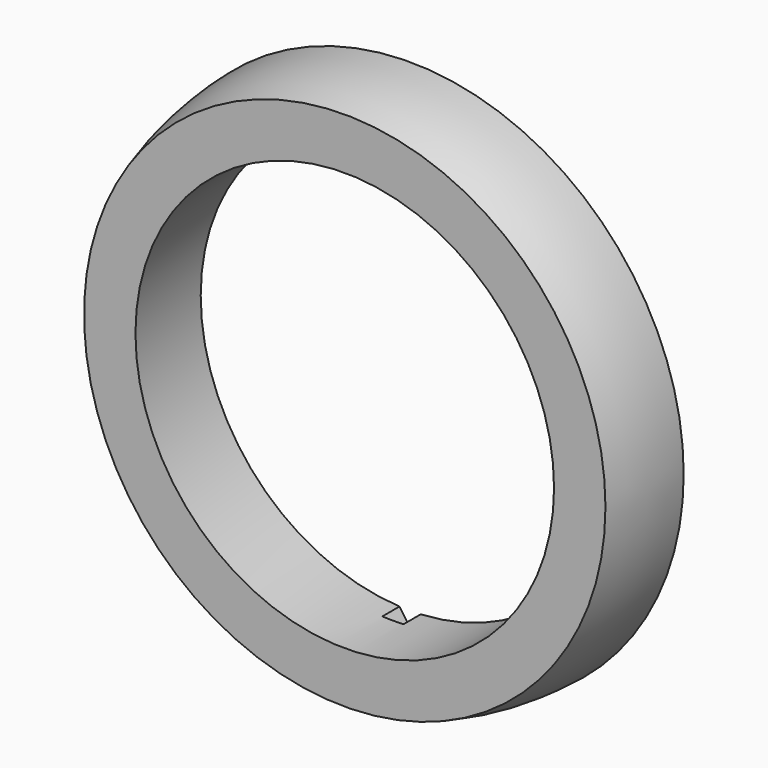
from build123d import *

# Parameters (mm, degrees)
F3_DEPTH = 10


with BuildPart() as f1:
    # F0 (on Top) → F1 (revolve)
    with BuildSketch(Plane.XY):
        with BuildLine():
            Line((97.4973875252, -38.8161949813), (121.4477377606, -38.8161949813))
            ThreePointArc((121.4477377606, -38.8161949813), (120.5697284263, -19.6675259883), (117.0955747366, -0.8161949813))
            Line((117.0955747366, -0.8161949813), (97.4973875252, -0.8161949813))
            Line((97.4973875252, -0.8161949813), (97.4973875252, -38.8161949813))
        make_face()
        with BuildLine():
            ThreePointArc((117.0955747366, -0.8161949813), (120.5697284263, -19.6675259883), (121.4477377606, -38.8161949813))
            ThreePointArc((121.4477377606, -38.8161949813), (125.914331396, -20.045726455), (127.4973875252, -0.8161949813))
            Line((127.4973875252, -0.8161949813), (117.0955747366, -0.8161949813))
        make_face()
    revolve(axis=Axis((0, 9.7614582628, 0), (0, -1, 0)))

    # F2 (on face) → F3 (cut)
    with BuildSketch(Plane(origin=(0, -0.8161949813, 0), x_dir=(-1, 0, 0), z_dir=(0, 1, 0))):
        with BuildLine():
            Line((-4.9983559861, -97.3691789617), (0.6029718567, -103.4572258853))
            Line((0.6029718567, -103.4572258853), (4.8713640334, -97.375614949))
            ThreePointArc((4.8713640334, -97.375614949), (2.4364429045, -97.4669396268), (0, -97.4973875252))
            ThreePointArc((0, -97.4973875252), (-2.5, -97.465330114), (-4.9983559861, -97.3691789617))
        make_face()
    extrude(amount=-F3_DEPTH, mode=Mode.SUBTRACT)


solid = f1.part
